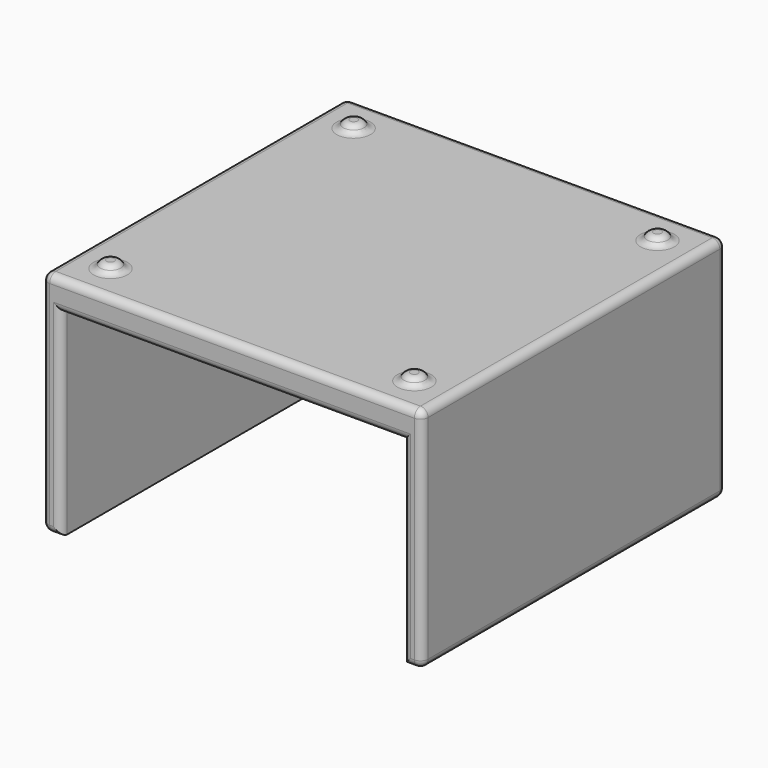
from build123d import *

# Parameters (mm, degrees)
F0_W          = 50
F0_H          = 30
F1_DEPTH      = 25
F1_DEPTH_BACK = 25
F2_W          = 45
F2_H          = 26
F3_DEPTH      = 47.5
F4_R          = 20.05
F5_DEPTH      = 3
F6_R          = 1.5
F7_DEPTH      = 1
F8_R          = 0.99999
F9_R          = 1


# Not quite as in the source:
# - a fillet or chamfer is up to 0.001 mm smaller than in the source, because OpenCascade refuses the exact size


with BuildPart() as f1:
    # F0 (on Front) → F1 (new body, two sides)
    with BuildSketch(Plane.XZ) as f1_sk:
        Rectangle(F0_W, F0_H)
    extrude(amount=F1_DEPTH)
    extrude(f1_sk.sketch, amount=-F1_DEPTH_BACK)

    # F2 (on face) → F3 (cut)
    with BuildSketch(Plane.XZ.offset(25)):
        with Locations((0, -2)):
            Rectangle(F2_W, F2_H)
    extrude(amount=-F3_DEPTH, mode=Mode.SUBTRACT)

    # F4 (on face) → F5 (cut)
    with BuildSketch(Plane(origin=(0, 0, 11), x_dir=(1, 0, 0), z_dir=(0, 0, -1))):
        Circle(F4_R)
    extrude(amount=-F5_DEPTH, mode=Mode.SUBTRACT)

    # F6 (on face) → F7 (join)
    with BuildSketch(Plane.XY.offset(15)):
        with Locations((-20, 20)):
            Circle(F6_R)
        with Locations((20, 20)):
            Circle(F6_R)
        with Locations((20, -20)):
            Circle(F6_R)
        with Locations((-20, -20)):
            Circle(F6_R)
    extrude(amount=F7_DEPTH)

    # F8 (radius 1 in the source; OpenCascade refuses exactly that, so slightly less here)
    f8_edges = [f1.edges().sort_by_distance(p)[0] for p in [
        (-21.5, -20, 16),
        (18.5, -20, 16),
        (18.5, 20, 16),
        (-21.5, 20, 16),
    ]]
    fillet(f8_edges, radius=F8_R)

    # F9
    f9_edges = [f1.edges().sort_by_distance(p)[0] for p in [
        (0, -25, 15),
        (25, 0, 15),
        (-25, 0, 15),
        (0, 25, 15),
        (18.5, -20, 15),
        (-21.5, -20, 15),
        (18.5, 20, 15),
        (-21.5, 20, 15),
        (-25, -25, 0),
        (25, -25, 0),
        (23.75, -25, -15),
        (22.5, -25, -2),
        (0, -25, 11),
        (-22.5, -25, -2),
        (-23.75, -25, -15),
        (25, 25, 0),
        (25, 0, -15),
        (0, 25, -15),
        (-25, 25, 0),
        (-25, 0, -15),
    ]]
    fillet(f9_edges, radius=F9_R)


solid = f1.part
